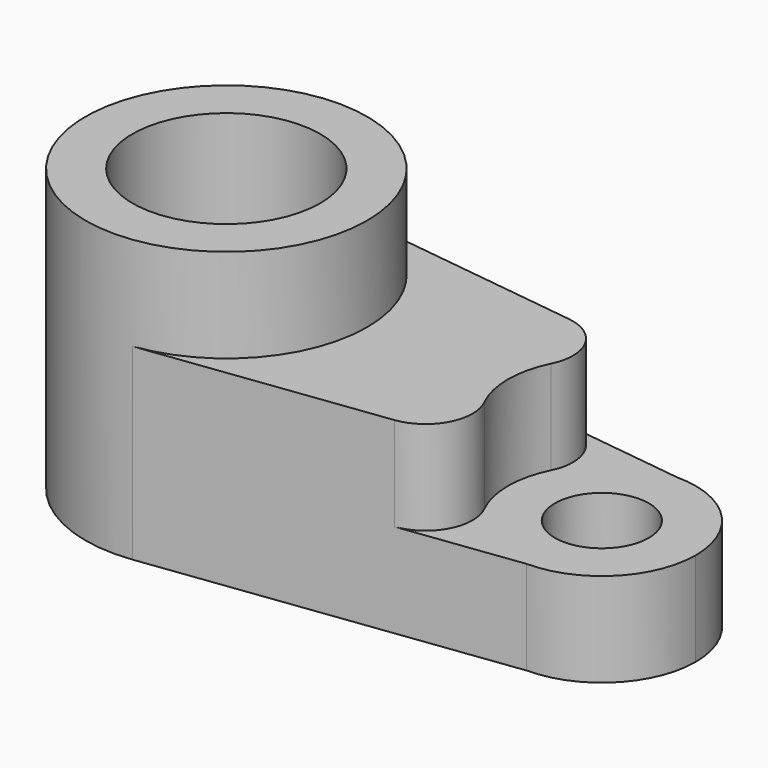
from build123d import *

# Parameters (mm, degrees)
F0_R     = 25.4
F1_DEPTH = 25.4
F0_R_2   = 12.7
F2_DEPTH = 50.8
F3_DEPTH = 76.2
F4_R     = 12.7


# Not quite as in the source:
# - a feature names something its author has since deleted; it is built from what else it names


with BuildPart() as f1:
    # F0 (on Top) → F1 (new body)
    with BuildSketch(Plane.XY):
        with BuildLine():
            ThreePointArc((4.8396572649, -37.7913709404), (28.6007075244, -25.1716016396), (38.1, 0))
            ThreePointArc((38.1, 0), (28.6007075244, 25.1716016396), (4.8396572649, 37.7913709404))
            ThreePointArc((4.8396572649, 37.7913709404), (-38.1, 0), (4.8396572649, -37.7913709404))
        make_face()
        Circle(F0_R, mode=Mode.SUBTRACT)
    extrude(amount=F1_DEPTH)



with BuildPart() as f1b:
    # F0 (on Top) → F1, piece 2 (new body)
    with BuildSketch(Plane.XY):
        with BuildLine():
            ThreePointArc((127, 0), (119.5605122421, 17.9605122421), (101.6, 25.4))
            ThreePointArc((101.6, 25.4), (76.2, 0), (101.6, -25.4))
            ThreePointArc((101.6, -25.4), (119.5605122421, -17.9605122421), (127, 0))
        make_face()
        with Locations((101.6, 0)):
            Circle(F0_R_2, mode=Mode.SUBTRACT)
    extrude(amount=F1_DEPTH)


with BuildPart() as f1_1:
    add(f1.part)

    add(f1b.part)  # F2 merges F1b
    # F0 (on Top) → F2 (join)
    with BuildSketch(Plane.XY):
        with BuildLine():
            ThreePointArc((4.8396572649, -37.7913709404), (28.6007075244, -25.1716016396), (38.1, 0))
            ThreePointArc((38.1, 0), (28.6007075244, 25.1716016396), (4.8396572649, 37.7913709404))
            ThreePointArc((4.8396572649, 37.7913709404), (-38.1, 0), (4.8396572649, -37.7913709404))
        make_face()
        Circle(F0_R, mode=Mode.SUBTRACT)
        with BuildLine():
            ThreePointArc((4.8396572649, 37.7913709404), (28.6007075244, 25.1716016396), (38.1, 0))
            ThreePointArc((38.1, 0), (28.6007075244, -25.1716016396), (4.8396572649, -37.7913709404))
            Line((4.8396572649, -37.7913709404), (101.6, -25.4))
            ThreePointArc((101.6, -25.4), (76.2, 0), (101.6, 25.4))
            Line((101.6, 25.4), (4.8396572649, 37.7913709404))
        make_face()
    extrude(amount=F2_DEPTH)

    # F0 (on Top) → F3 (join)
    with BuildSketch(Plane.XY):
        with BuildLine():
            ThreePointArc((4.8396572649, -37.7913709404), (28.6007075244, -25.1716016396), (38.1, 0))
            ThreePointArc((38.1, 0), (28.6007075244, 25.1716016396), (4.8396572649, 37.7913709404))
            ThreePointArc((4.8396572649, 37.7913709404), (-38.1, 0), (4.8396572649, -37.7913709404))
        make_face()
        Circle(F0_R, mode=Mode.SUBTRACT)
    extrude(amount=F3_DEPTH)

    # F4
    f4_edges = [f1_1.edges().sort_by_distance(p)[0] for p in [
        (101.6, -25.4, 38.1),
        (101.6, 25.4, 38.1),
    ]]
    fillet(f4_edges, radius=F4_R)


solid = f1_1.part
